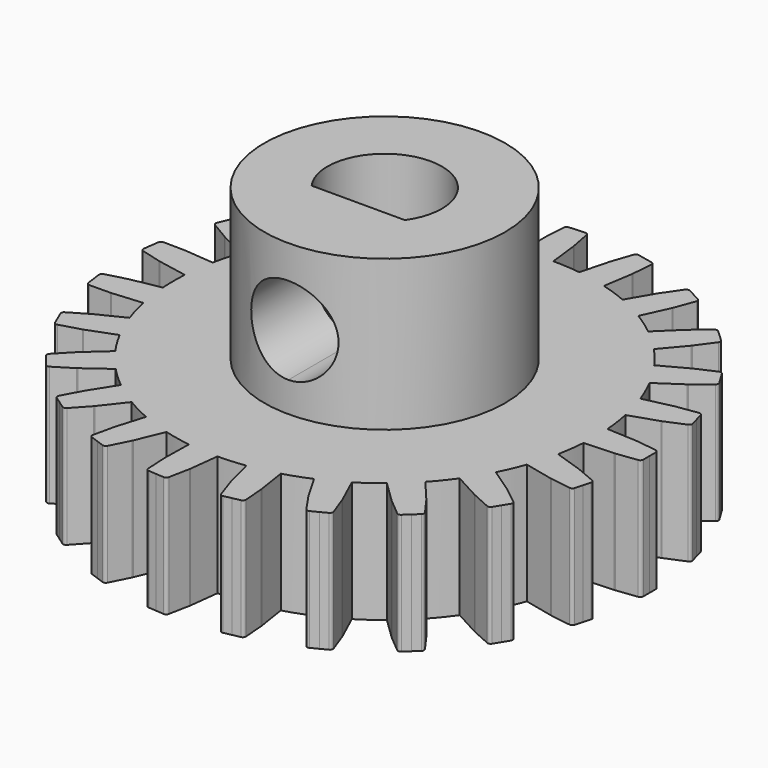
from build123d import *

# Parameters (mm, degrees)
F0_R     = 4
F2_DEPTH = 7
F3_DEPTH = 2
F4_DEPTH = 2
F5_DEPTH = 2
F6_COUNT = 23
F9_DEPTH = 7.88


# Not quite as in the source:
# - after a boolean that leaves OpenCascade's solid faulty, fix() repairs it
# - a feature names something its author has since deleted; it is built from what else it names


with BuildPart() as f2:
    # F0 (on Top) → F2 (new body)
    with BuildSketch(Plane.XY):
        Circle(F0_R)
        with BuildLine():
            ThreePointArc((-1.5491933385, -1.1), (-0.5772922383, 1.8101750389), (1.9, 0))
            ThreePointArc((1.9, 0), (1.8101750389, -0.5772922383), (1.5491933385, -1.1))
            ThreePointArc((1.5491933385, -1.1), (0, -1.9), (-1.5491933385, -1.1))
        make_face(mode=Mode.SUBTRACT)
        with BuildLine():
            Line((1.5491933385, -1.1), (-1.5491933385, -1.1))
            ThreePointArc((-1.5491933385, -1.1), (0, -1.9), (1.5491933385, -1.1))
        make_face()
    extrude(amount=F2_DEPTH)

    # F0 (on Top) → F3 (join)
    with BuildSketch(Plane.XY):
        Circle(F0_R)
        with BuildLine():
            ThreePointArc((-1.5491933385, -1.1), (-0.5772922383, 1.8101750389), (1.9, 0))
            ThreePointArc((1.9, 0), (1.8101750389, -0.5772922383), (1.5491933385, -1.1))
            ThreePointArc((1.5491933385, -1.1), (0, -1.9), (-1.5491933385, -1.1))
        make_face(mode=Mode.SUBTRACT)
    extrude(amount=-F3_DEPTH)

    # F0 (on Top) → F4 (join, symmetric)
    with BuildSketch(Plane.XY):
        with BuildLine():
            Line((-0.4987182067, 6.9642860474), (-0.9974457174, 6.9285714286))
            ThreePointArc((-0.9974457174, 6.9285714286), (0.5, -6.9821200219), (0, 7))
            Line((0, 7), (-0.4987182067, 6.9642860474))
        make_face()
        Circle(F0_R, mode=Mode.SUBTRACT)
    extrude(amount=F4_DEPTH, both=True)

    add(f2.part.fix(), mode=Mode.REPLACE)



with BuildPart() as f5:
    # F0 (on Top) → F5 (new body, symmetric)
    with BuildSketch(Plane.XY):
        with BuildLine():
            Line((-1.0143579612, 7.9110673661), (-0.9974457174, 6.9285714286))
            Line((-0.9974457174, 6.9285714286), (-0.4987182067, 6.9642860474))
            Line((-0.4987182067, 6.9642860474), (-0.5656930017, 7.9598762295))
            Line((-0.5656930017, 7.9598762295), (-1.0143315548, 7.9296956636))
            ThreePointArc((-1.0143315548, 7.9296956636), (-1.014431519, 7.9203816378), (-1.0143579612, 7.9110673661))
        make_face()
        with BuildLine():
            Line((-0.4987182067, 6.9642860474), (0, 7))
            Line((0, 7), (-0.1145355074, 7.9716517958))
            ThreePointArc((-0.1145355074, 7.9716517958), (-0.115708533, 7.9808660507), (-0.1170525242, 7.9900569249))
            Line((-0.1170525242, 7.9900569249), (-0.5656930017, 7.9598762295))
            Line((-0.5656930017, 7.9598762295), (-0.4987182067, 6.9642860474))
        make_face()
        with BuildLine():
            Line((-1.0143315548, 7.9296956636), (-0.5656930017, 7.9598762295))
            Line((-0.5656930017, 7.9598762295), (-0.6193888, 8.7580721712))
            Line((-0.6193888, 8.7580721712), (-0.8805203765, 8.7405054714))
            ThreePointArc((-0.8805203765, 8.7405054714), (-0.9448712377, 8.7110877363), (-0.9736449414, 8.6464463374))
            Line((-0.9736449414, 8.6464463374), (-1.0136147202, 7.9482496599))
            ThreePointArc((-1.0136147202, 7.9482496599), (-1.0140592718, 7.9389759895), (-1.0143315548, 7.9296956636))
        make_face()
        with BuildLine():
            Line((-0.6193888, 8.7580721712), (-0.5656930017, 7.9598762295))
            Line((-0.5656930017, 7.9598762295), (-0.1170525242, 7.9900569249))
            ThreePointArc((-0.1170525242, 7.9900569249), (-0.1185618327, 7.9991915846), (-0.120240022, 8.0082967315))
            Line((-0.120240022, 8.0082967315), (-0.253373745, 8.694900025))
            ThreePointArc((-0.253373745, 8.694900025), (-0.2905460548, 8.75510514), (-0.3582572236, 8.7756388709))
            Line((-0.3582572236, 8.7756388709), (-0.6193888, 8.7580721712))
        make_face()
    extrude(amount=F5_DEPTH, both=True)


with BuildPart() as f2_1:
    add(f2.part)

    add(f5.part)  # F6 merges F5
    # F6: F5 ×23 about axis
    f6_axis = Axis((0, 0, 13.3862942457), (0, 0, 1))
    for i in range(1, F6_COUNT):
        add(f5.part.rotate(f6_axis, i * 360 / F6_COUNT))

    # F8 (on offset) → F9 (cut)
    with BuildSketch(Plane.XZ.offset(8.8)):
        with BuildLine():
            ThreePointArc((0, 3.0039259397), (1.0253048327, 3.428621107), (1.45, 4.4539259397))
            ThreePointArc((1.45, 4.4539259397), (1.0253048327, 5.4792307725), (0, 5.9039259397))
            Line((0, 5.9039259397), (0, 3.0039259397))
        make_face()
        with BuildLine():
            Line((0, 3.0039259397), (0, 5.9039259397))
            ThreePointArc((0, 5.9039259397), (-1.45, 4.4539259397), (0, 3.0039259397))
        make_face()
    extrude(amount=-F9_DEPTH, mode=Mode.SUBTRACT)


solid = f2_1.part
